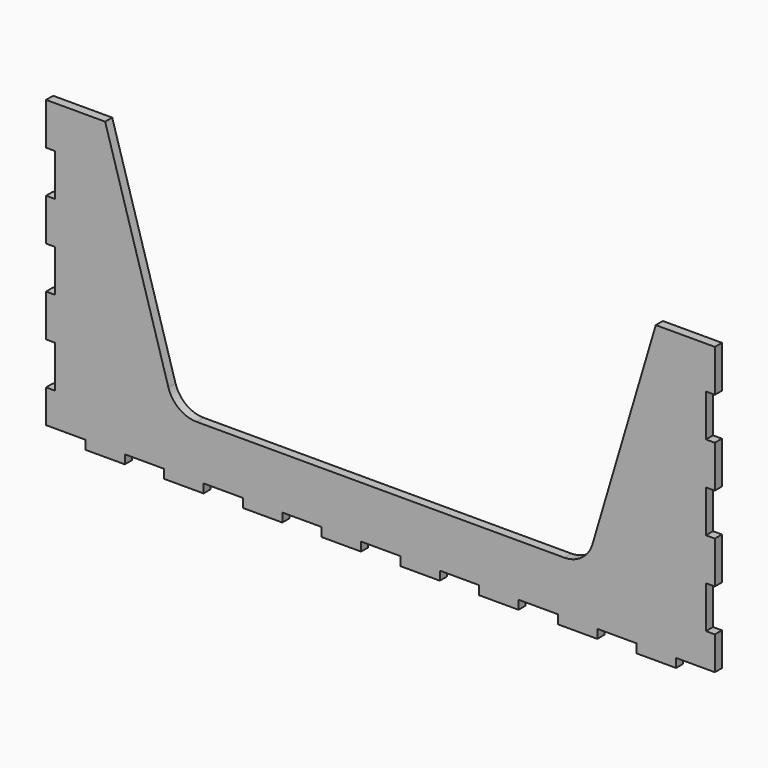
from build123d import *

# Parameters (mm, degrees)
F1_DEPTH = 3


# Not quite as in the source:
# - ends of sketch curves that miss each other by under 0.0002 mm in the source are joined


with BuildPart() as f1:
    # F0 (on Front) → F1 (new body)
    with BuildSketch(Plane.XZ):
        with BuildLine():
            Line((60.097833329, -50), (73.431166662, -50))
            Line((73.431166662, -50), (73.431166662, -47))
            Line((73.431166662, -47), (86.7645, -47))
            Line((86.7645, -47), (86.7645, -50.0000007451))
            Line((86.7645, -50.0000007451), (100.097833333, -50.0000007451))
            Line((100.097833333, -50.0000007451), (100.097833333, -47.0000007451))
            Line((100.097833333, -47.0000007451), (113.2355, -47.0000007451))
            Line((113.2355, -47.0000007451), (113.2355, -35.714285716))
            Line((113.2355, -35.714285716), (110.2355, -35.714285716))
            Line((110.2355, -35.714285716), (110.2355, -21.42857143))
            Line((110.2355, -21.42857143), (113.2355, -21.42857143))
            Line((113.2355, -21.42857143), (113.2355, -7.142857144))
            Line((113.2355, -7.142857144), (110.2355, -7.142857144))
            Line((110.2355, -7.142857144), (110.2355, 7.142857142))
            Line((110.2355, 7.142857142), (113.2355, 7.142857142))
            Line((113.2355, 7.142857142), (113.2355, 21.428571428))
            Line((113.2355, 21.428571428), (110.2355, 21.428571428))
            Line((110.2355, 21.428571428), (110.2355, 35.714285714))
            Line((110.2355, 35.714285714), (113.2355, 35.714285714))
            Line((113.2355, 35.714285714), (113.2355, 50))
            Line((113.2355, 50), (93.2355, 50))
            Line((93.2355, 50), (71.8119617716, -22.2537644208))
            ThreePointArc((71.8119617716, -22.2537644208), (68.2066991862, -27.4243868361), (62.2245235205, -29.4110495597))
            Line((62.2245235205, -29.4110495597), (0, -29.4110495597))
            Line((0, -29.4110495597), (-62.2245235205, -29.4110495597))
            ThreePointArc((-62.2245235205, -29.4110495597), (-68.2066991862, -27.4243868361), (-71.8119617716, -22.2537644208))
            Line((-71.8119617716, -22.2537644208), (-93.2355, 50))
            Line((-93.2355, 50), (-113.2355, 50))
            Line((-113.2355, 50), (-113.2355, 35.714285714))
            Line((-113.2355, 35.714285714), (-110.2355, 35.714285714))
            Line((-110.2355, 35.714285714), (-110.2355, 21.428571428))
            Line((-110.2355, 21.428571428), (-113.2355, 21.428571428))
            Line((-113.2355, 21.428571428), (-113.2355, 7.142857142))
            Line((-113.2355, 7.142857142), (-110.2355, 7.142857142))
            Line((-110.2355, 7.142857142), (-110.2355, -7.142857144))
            Line((-110.2355, -7.142857144), (-113.2355, -7.142857144))
            Line((-113.2355, -7.142857144), (-113.2355, -21.42857143))
            Line((-113.2355, -21.42857143), (-110.2355, -21.42857143))
            Line((-110.2355, -21.42857143), (-110.2355, -35.714285716))
            Line((-110.2355, -35.714285716), (-113.2355, -35.714285716))
            Line((-113.2355, -35.714285716), (-113.2355, -47))
            Line((-113.2355, -47), (-99.902166667, -47))
            Line((-99.902166667, -47), (-99.902166667, -50))
            Line((-99.902166667, -50), (-86.568833334, -50))
            Line((-86.568833334, -50), (-86.568833334, -47))
            Line((-86.568833334, -47), (-73.235500001, -47))
            Line((-73.235500001, -47), (-73.235500001, -50))
            Line((-73.235500001, -50), (-59.902166668, -50))
            Line((-59.902166668, -50), (-59.902166668, -47))
            Line((-59.902166668, -47), (-46.568833335, -47))
            Line((-46.568833335, -47), (-46.568833335, -50))
            Line((-46.568833335, -50), (-33.235500002, -50))
            Line((-33.235500002, -50), (-33.235500002, -47))
            Line((-33.235500002, -47), (-19.902166669, -47))
            Line((-19.902166669, -47), (-19.902166669, -50))
            Line((-19.902166669, -50), (-6.568833336, -50))
            Line((-6.568833336, -50), (-6.568833336, -47))
            Line((-6.568833336, -47), (6.764499997, -47))
            Line((6.764499997, -47), (6.764499997, -50))
            Line((6.764499997, -50), (20.09783333, -50))
            Line((20.09783333, -50), (20.09783333, -47))
            Line((20.09783333, -47), (33.431166663, -47))
            Line((33.431166663, -47), (33.431166663, -50))
            Line((33.431166663, -50), (46.764499996, -50))
            Line((46.764499996, -50), (46.764499996, -47))
            Line((46.764499996, -47), (60.097833329, -47))
            Line((60.097833329, -47), (60.097833329, -50))
        make_face()
    extrude(amount=F1_DEPTH)


solid = f1.part
